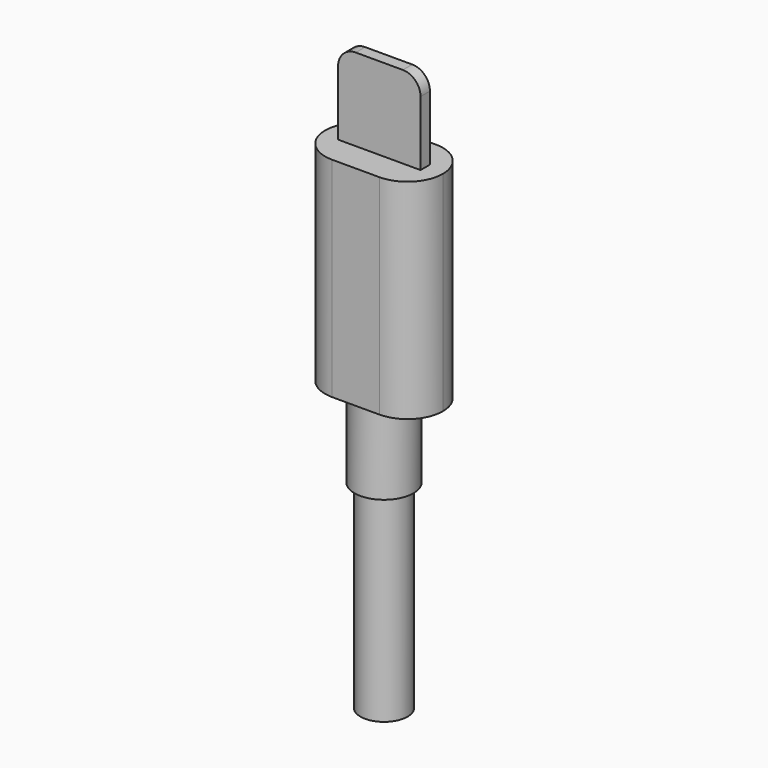
from build123d import *

# Parameters (mm, degrees)
F1_DEPTH = 7.62
F2_DEPTH = 1.27
F0_W     = 5.08
F0_H     = 42.841874063
F5_R     = 7.61999


# Not quite as in the source:
# - a fillet or chamfer is up to 0.001 mm smaller than in the source, because OpenCascade refuses the exact size


with BuildPart() as f1:
    # F0 (on Front) → F1 (new body, symmetric)
    with BuildSketch(Plane.XZ):
        Polygon((-45.6967013121, 20.0940572381), (-39.3467013121, 20.0940572381), (-39.3467013121, 65.1790572381), (-43.1567013121, 65.1790572381), (-60.9367013121, 65.1790572381), (-64.7467013121, 65.1790572381), (-64.7467013121, 20.0940572381), (-58.3967013121, 20.0940572381), (-52.0467013121, 20.0940572381), align=None)
    extrude(amount=F1_DEPTH, both=True)

    # F0 (on Front) → F2 (join, symmetric)
    with BuildSketch(Plane.XZ):
        with BuildLine():
            Line((-60.9367013121, 65.1790572381), (-43.1567013121, 65.1790572381))
            Line((-43.1567013121, 65.1790572381), (-43.1567013121, 79.1490572381))
            ThreePointArc((-43.1567013121, 79.1490572381), (-44.2726244757, 81.8431340744), (-46.9667013121, 82.9590572381))
            Line((-46.9667013121, 82.9590572381), (-57.1267013121, 82.9590572381))
            ThreePointArc((-57.1267013121, 82.9590572381), (-59.8207781484, 81.8431340744), (-60.9367013121, 79.1490572381))
            Line((-60.9367013121, 79.1490572381), (-60.9367013121, 65.1790572381))
        make_face()
    extrude(amount=F2_DEPTH, both=True)

    # F0 (on Front) → F3 (revolve)
    with BuildSketch(Plane.XZ):
        Polygon((-52.0467013121, 2.457652241), (-52.0467013121, 20.0940572381), (-58.3967013121, 20.0940572381), (-58.3967013121, 2.457652241), (-57.1267013121, 2.457652241), align=None)
    revolve(axis=Axis((-52.0467013121, 0, -10.145082292), (0, 0, -1)))

    # F0 (on Front) → F4 (revolve)
    with BuildSketch(Plane.XZ):
        with Locations((-54.5867013121, -18.9632847905)):
            Rectangle(F0_W, F0_H)
    revolve(axis=Axis((-52.0467013121, 0, -10.145082292), (0, 0, -1)))

    # F5 (radius 7.62 in the source; OpenCascade refuses exactly that, so slightly less here)
    f5_edges = [f1.edges().sort_by_distance(p)[0] for p in [
        (-39.346701, 7.62, 42.636557),
        (-64.746701, 7.62, 42.636557),
        (-64.746701, -7.62, 42.636557),
        (-39.346701, -7.62, 42.636557),
    ]]
    fillet(f5_edges, radius=F5_R)


solid = f1.part
